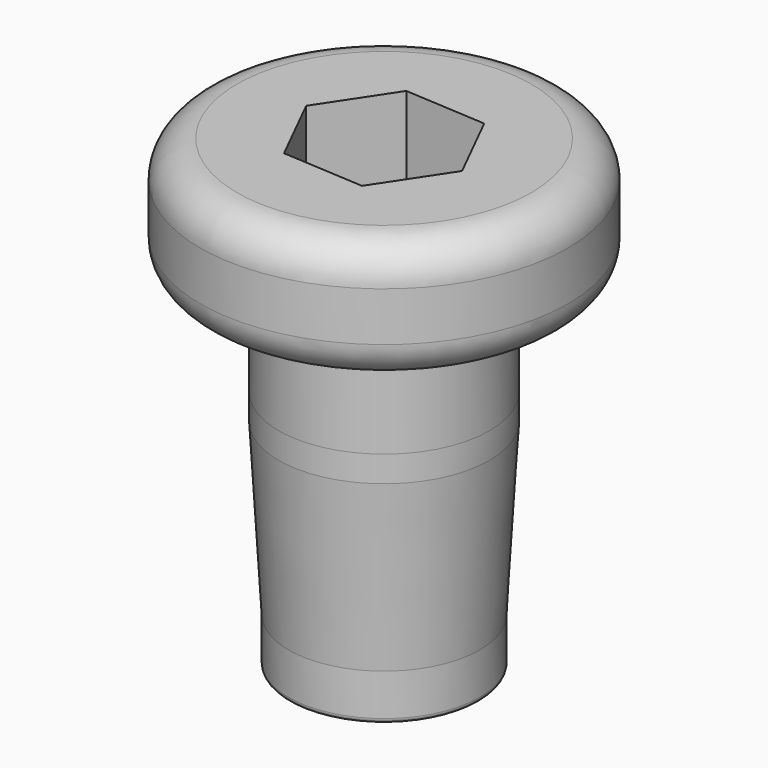
from build123d import *

# Parameters (mm, degrees)
F0_R         = 3.9
F2_DEPTH     = 14
F3_R         = 7.5
F4_DEPTH     = 5
F6_R         = 4.3
F7_DEPTH     = 4.1
F1_R         = 1.5693660879
F8_DEPTH     = 23.4
F9_DEPTH     = 15.5
F10_R        = 0.2
F11_S5_R     = 4.3
F11_T6_DEPTH = 9
F12_R        = 1.5
F13_R        = 1.5


# Not quite as in the source:
# - a fillet or chamfer that OpenCascade refuses, or shapes differently, is made with other operations: its cross-section is extruded or revolved along the edge and cut away or added


with BuildPart() as f2:
    # F0 (on Top) → F2 (new body)
    with BuildSketch(Plane.XY):
        with Locations((-41.4718948305, -26.0946750641)):
            Circle(F0_R)
    extrude(amount=F2_DEPTH)

    # F3 (on face) → F4 (join)
    with BuildSketch(Plane.XY.offset(14)):
        with Locations((-41.4718948305, -26.0946750641)):
            Circle(F3_R)
    extrude(amount=F4_DEPTH)

    # F6 (on face) → F7 (join)
    with BuildSketch(Plane(origin=(0, 0, 14), x_dir=(1, 0, 0), z_dir=(0, 0, -1))):
        with Locations((-41.4718948305, 26.0946750641)):
            Circle(F6_R)
    extrude(amount=F7_DEPTH)

    # F1 (on Top) → F8 (cut)
    with BuildSketch(Plane.XY):
        with Locations((-41.495975107, -26.0728988796)):
            Circle(F1_R)
    extrude(amount=F8_DEPTH, mode=Mode.SUBTRACT)

    # F5 (on face) → F9 (cut)
    with BuildSketch(Plane.XY.offset(19)):
        Polygon((-39.9783341683, -29.0917753096), (-38.1295495491, -26.2997637113), (-39.6231102113, -23.3026634658), (-42.9654554927, -23.0975748186), (-44.8142401119, -25.8895864169), (-43.3206794497, -28.8866866624), align=None)
    extrude(amount=-F9_DEPTH, mode=Mode.SUBTRACT)

    # F10
    f10_edges = [f2.edges().sort_by_distance(p)[0] for p in [
        (-45.371895, -26.094675, 0),
    ]]
    fillet(f10_edges, radius=F10_R)

    # F11: chamfer of 8 x 0.4612770977 on 1 edges, made by hand


with BuildPart() as f11_tool2:
    # F11_s3 → F11_t4 (revolve)
    with BuildSketch(Plane.XZ.offset(26.0946750641)):
        Polygon((-37.5718948305, 1.9), (-37.1106177328, 9.9), (-37.5718948305, 9.9), align=None)
    revolve(axis=Axis((-41.4718948305, -26.0946750641, 9.9), (0, 0, -1)))

    # F11_s5 → F11_t6 (intersect, symmetric)
    with BuildSketch(Plane.XY.offset(5.9)):
        with Locations((-41.4718948305, -26.0946750641)):
            Circle(F11_S5_R)
    extrude(amount=F11_T6_DEPTH, both=True, mode=Mode.INTERSECT)


with BuildPart() as f2_1:
    add(f2.part)

    # F11_t1: union F11_tool2
    add(f11_tool2.part)

    # F12
    f12_edges = [f2_1.edges().sort_by_distance(p)[0] for p in [
        (-48.971895, -26.094675, 14),
    ]]
    fillet(f12_edges, radius=F12_R)

    # F13
    f13_edges = [f2_1.edges().sort_by_distance(p)[0] for p in [
        (-48.971895, -26.094675, 19),
    ]]
    fillet(f13_edges, radius=F13_R)


solid = f2_1.part
